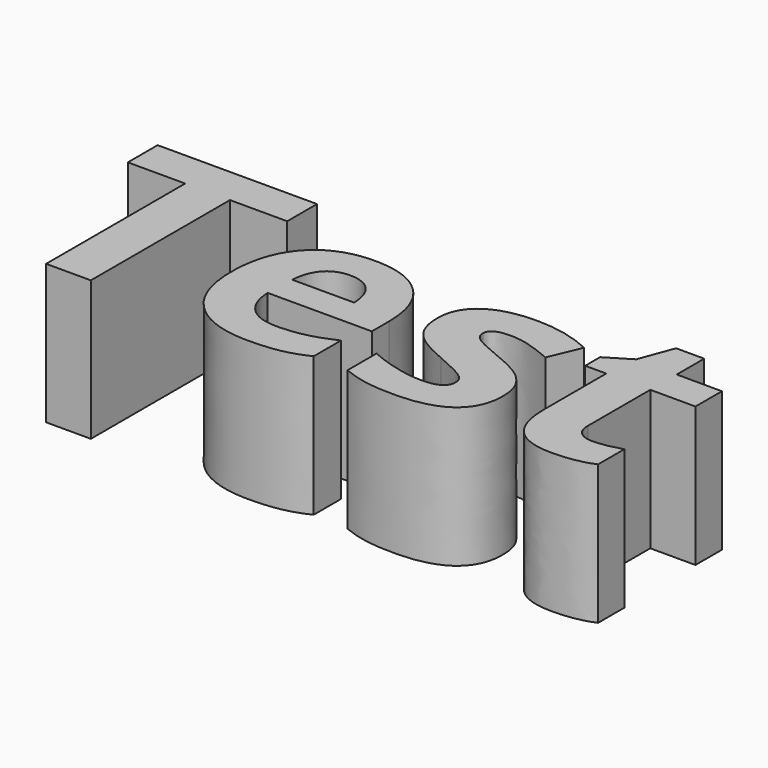
from build123d import *

# Parameters (mm, degrees)
F0_TEXT_SIZE = 52.973933311
F1_DEPTH     = 25


# Not quite as in the source:
# - Text() gives the source's letters only with a copy of the font that has no kerning and outlines rounded to 1/6400 em; it was checked with that copy


with BuildPart() as f1:
    # F0 (on Top) → F1 (new body)
    with BuildSketch(Plane.XY):
        with Locations((0, -38.1412319839)):
            Text('Test', F0_TEXT_SIZE, font='Open Sans', font_style=FontStyle.BOLD, text_align=(TextAlign.LEFT, TextAlign.BOTTOM))
    extrude(amount=F1_DEPTH)


solid = f1.part
